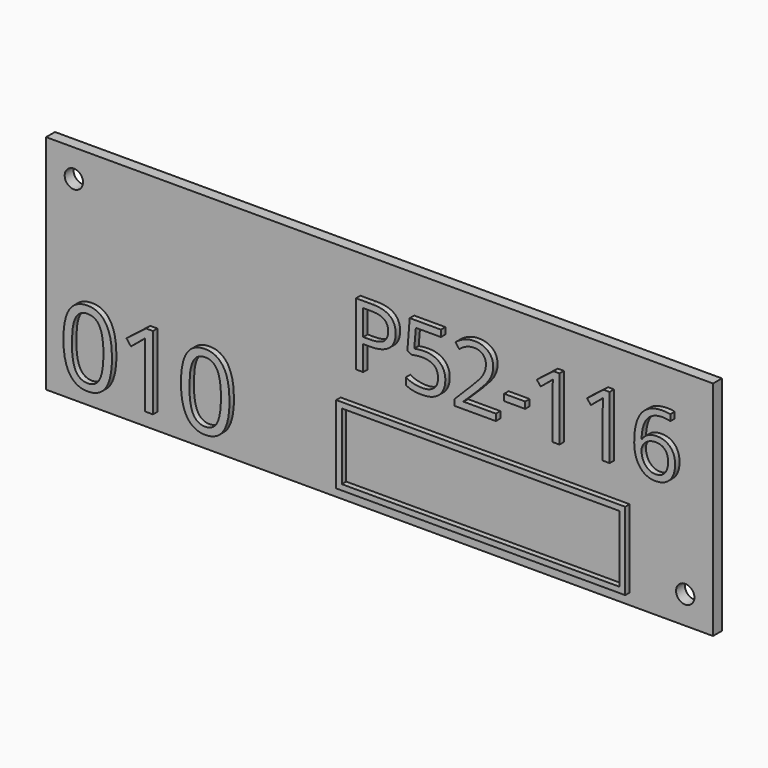
from build123d import *

# Parameters (mm, degrees)
F0_W         = 120
F0_H         = 40
F1_DEPTH     = 2
F3_D         = 3.3
F4_TEXT_SIZE = 15.7959687371
F5_DEPTH     = 1
F6_TEXT_SIZE = 18.4937691891
F7_DEPTH     = 1
F8_W         = 52
F8_H         = 14
F8_W_2       = 49.99999962
F8_H_2       = 11.99999962
F9_DEPTH     = 1


# Not quite as in the source:
# - Text() gives the source's letters only with a copy of the font that has no kerning and outlines rounded to 1/6400 em; it was checked with that copy


with BuildPart() as f1:
    # F0 (on Front) → F1 (new body)
    with BuildSketch(Plane.XZ):
        Rectangle(F0_W, F0_H)
    extrude(amount=F1_DEPTH)

    # F3 (through all)
    with Locations(Plane.XZ.offset(2)):
        with Locations((-55, 15), (55, -15)):
            Hole(F3_D / 2)

    # F4 (on face) → F5 (join)
    with BuildSketch(Plane.XZ.offset(2)):
        with Locations((-5, 2)):
            Text('P52-116', F4_TEXT_SIZE, font='Open Sans', text_align=(TextAlign.LEFT, TextAlign.BOTTOM))
    extrude(amount=F5_DEPTH)

    # F6 (on face) → F7 (join)
    with BuildSketch(Plane.XZ.offset(2)):
        with Locations((-57, -17)):
            Text('010', F6_TEXT_SIZE, font='Open Sans', text_align=(TextAlign.LEFT, TextAlign.BOTTOM))
    extrude(amount=F7_DEPTH)

    # F8 (on face) → F9 (join)
    with BuildSketch(Plane.XZ.offset(2)):
        with Locations((19, -11)):
            Rectangle(F8_W, F8_H)
        with Locations((19, -11)):
            Rectangle(F8_W_2, F8_H_2, mode=Mode.SUBTRACT)
    extrude(amount=F9_DEPTH)


solid = f1.part
